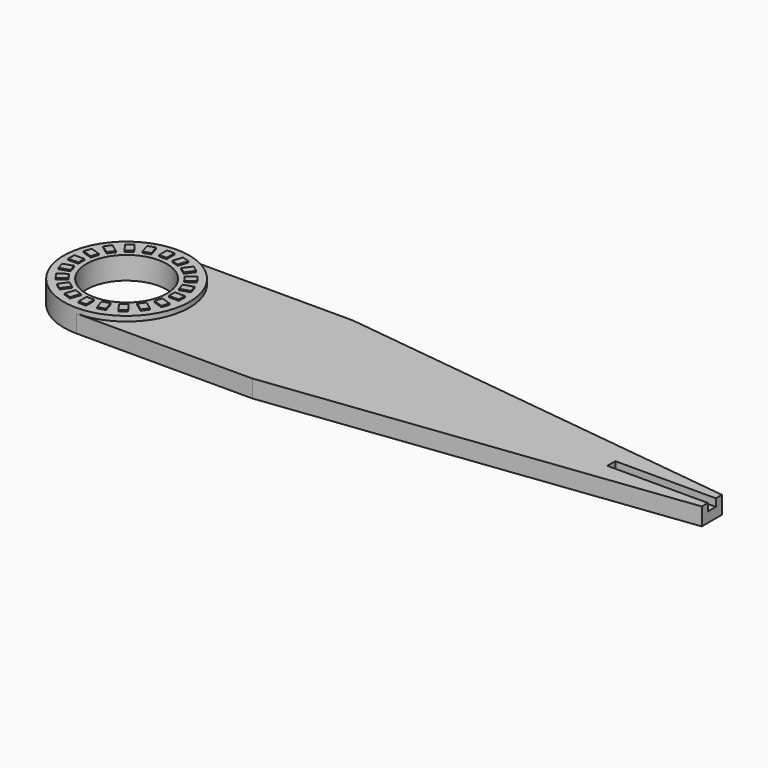
from build123d import *

# Parameters (mm, degrees)
F0_R         = 8
F1_DEPTH     = 3.5
F2_R         = 12.5
F2_R_2       = 8
F3_DEPTH     = 1
F4_W         = 1.5
F4_H         = 2
F4_W_2       = 2
F4_H_2       = 1.5
F5_DEPTH     = 0.25
F6_W         = 20
F6_H         = 2
F7_DEPTH     = 1.5
F9_TEXT_SIZE = 25.0048837664
F10_DEPTH    = 1.5


# Not quite as in the source:
# - Text() gives the source's letters only with a copy of the font that has no kerning and outlines rounded to 1/6400 em; it was checked with that copy


with BuildPart() as f1:
    # F0 (on Top) → F1 (new body)
    with BuildSketch(Plane.XY):
        with BuildLine():
            ThreePointArc((0, -12.5), (8.8388347648, -8.8388347648), (12.5, 0))
            ThreePointArc((12.5, 0), (8.8388347648, 8.8388347648), (0, 12.5))
            ThreePointArc((0, 12.5), (-12.5, 0), (0, -12.5))
        make_face()
        Circle(F0_R, mode=Mode.SUBTRACT)
        with BuildLine():
            ThreePointArc((0, 12.5), (8.8388347648, 8.8388347648), (12.5, 0))
            ThreePointArc((12.5, 0), (8.8388347648, -8.8388347648), (0, -12.5))
            Line((0, -12.5), (35, -12.5))
            Line((35, -12.5), (116.3887844346, -2.5067138408))
            Line((116.3887844346, -2.5067138408), (116.3887844346, 2.5067138408))
            Line((116.3887844346, 2.5067138408), (35, 12.5))
            Line((35, 12.5), (0, 12.5))
        make_face()
    extrude(amount=F1_DEPTH)

    # F2 (on face) → F3 (join)
    with BuildSketch(Plane.XY.offset(3.5)):
        Circle(F2_R)
        Circle(F2_R_2, mode=Mode.SUBTRACT)
    extrude(amount=F3_DEPTH)

    # F4 (on face) → F5 (join)
    with BuildSketch(Plane.XY.offset(4.5)):
        with Locations((0, 10)):
            Rectangle(F4_W, F4_H)
        Polygon((-2.6858945509, 10.693384425), (-4.1124793253, 10.2298589335), (-3.4944453366, 8.3277459009), (-2.0678605622, 8.7912713924), align=None)
        Polygon((-5.8588750294, 9.3400258773), (-7.072400521, 8.4583479989), (-5.8968300164, 6.8403140102), (-4.6833045249, 7.7219918886), align=None)
        Polygon((-8.4583479989, 7.072400521), (-9.3400258773, 5.8588750294), (-7.7219918886, 4.6833045249), (-6.8403140102, 5.8968300164), align=None)
        Polygon((-10.2298589335, 4.1124793253), (-10.693384425, 2.6858945509), (-8.7912713924, 2.0678605622), (-8.3277459009, 3.4944453366), align=None)
        with Locations((-10, 0)):
            Rectangle(F4_W_2, F4_H_2)
        Polygon((-10.693384425, -2.6858945509), (-10.2298589335, -4.1124793253), (-8.3277459009, -3.4944453366), (-8.7912713924, -2.0678605622), align=None)
        Polygon((-9.3400258773, -5.8588750294), (-8.4583479989, -7.072400521), (-6.8403140102, -5.8968300164), (-7.7219918886, -4.6833045249), align=None)
        Polygon((-7.072400521, -8.4583479989), (-5.8588750294, -9.3400258773), (-4.6833045249, -7.7219918886), (-5.8968300164, -6.8403140102), align=None)
        Polygon((-4.1124793253, -10.2298589335), (-2.6858945509, -10.693384425), (-2.0678605622, -8.7912713924), (-3.4944453366, -8.3277459009), align=None)
        with Locations((0, -10)):
            Rectangle(F4_W, F4_H)
        Polygon((2.6858945509, -10.693384425), (4.1124793253, -10.2298589335), (3.4944453366, -8.3277459009), (2.0678605622, -8.7912713924), align=None)
        Polygon((5.8588750294, -9.3400258773), (7.072400521, -8.4583479989), (5.8968300164, -6.8403140102), (4.6833045249, -7.7219918886), align=None)
        Polygon((8.4583479989, -7.072400521), (9.3400258773, -5.8588750294), (7.7219918886, -4.6833045249), (6.8403140102, -5.8968300164), align=None)
        Polygon((10.2298589335, -4.1124793253), (10.693384425, -2.6858945509), (8.7912713924, -2.0678605622), (8.3277459009, -3.4944453366), align=None)
        with Locations((10, 0)):
            Rectangle(F4_W_2, F4_H_2)
        Polygon((10.693384425, 2.6858945509), (10.2298589335, 4.1124793253), (8.3277459009, 3.4944453366), (8.7912713924, 2.0678605622), align=None)
        Polygon((9.3400258773, 5.8588750294), (8.4583479989, 7.072400521), (6.8403140102, 5.8968300164), (7.7219918886, 4.6833045249), align=None)
        Polygon((7.072400521, 8.4583479989), (5.8588750294, 9.3400258773), (4.6833045249, 7.7219918886), (5.8968300164, 6.8403140102), align=None)
        Polygon((4.1124793253, 10.2298589335), (2.6858945509, 10.693384425), (2.0678605622, 8.7912713924), (3.4944453366, 8.3277459009), align=None)
    extrude(amount=F5_DEPTH)

    # F6 (on face) → F7 (cut)
    with BuildSketch(Plane.XY.offset(3.5)):
        with Locations((106.3887844346, 0.0067138408)):
            Rectangle(F6_W, F6_H)
    extrude(amount=-F7_DEPTH, mode=Mode.SUBTRACT)

    # F9 (on line) → F10 (cut)
    with BuildSketch(Plane(origin=(0, 0, 0), x_dir=(1, 0, 0), z_dir=(0, 0, -1))):
        with Locations((12, -9.0017581559)):
            Text('Al', F9_TEXT_SIZE, font='Open Sans', text_align=(TextAlign.LEFT, TextAlign.BOTTOM))
    extrude(amount=-F10_DEPTH, mode=Mode.SUBTRACT)


solid = f1.part
